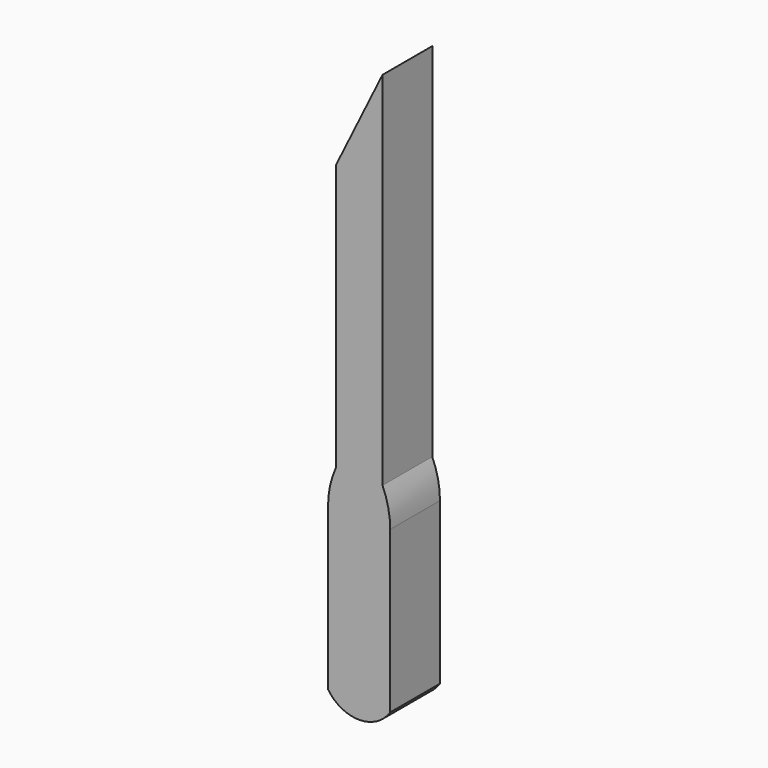
from build123d import *

# Parameters (mm, degrees)
F1_DEPTH    = 3.5
F2_T1_DEPTH = 13.6927447268
F2_T3_DEPTH = 13.6880389421


# Not quite as in the source:
# - a fillet or chamfer that OpenCascade refuses, or shapes differently, is made with other operations: its cross-section is extruded or revolved along the edge and cut away or added


with BuildPart() as f1:
    # F0 (on Front) → F1 (new body)
    with BuildSketch(Plane.XZ):
        with BuildLine():
            Line((-12.9772726037, -35.7954576612), (-16.4772726037, -35.7954576612))
            ThreePointArc((-16.4772726037, -35.7954576612), (-14.7272726037, -36.734376134), (-12.9772726037, -35.7954576612))
        make_face()
        Polygon((-16.0428304225, -9.6928073466), (-16.0428304225, -24.6928073466), (-13.4112946689, -24.6928073466), (-13.4112946689, -4.3468838558), align=None)
        Polygon((-16.4772726037, -24.6928073466), (-16.4772726037, -35.7954576612), (-12.9772726037, -35.7954576612), (-12.9772726037, -24.6928073466), (-13.4112946689, -24.6928073466), (-16.0428304225, -24.6928073466), align=None)
    extrude(amount=F1_DEPTH)

    # F2: fillet of radius 5 on 2 edges, made by hand

    # F2_s2 → F2_t1 (cut)
    with BuildSketch(Plane.XZ.offset(-5.0963723634)):
        with BuildLine():
            ThreePointArc((-16.0428304225, -24.6928073466), (-16.3674560917, -25.6891924599), (-16.4772726037, -26.7313562919))
            Line((-16.4772726037, -26.7313562919), (-16.4772726037, -24.6928073466))
            Line((-16.4772726037, -24.6928073466), (-16.0428304225, -24.6928073466))
        make_face()
    extrude(amount=F2_T1_DEPTH, mode=Mode.SUBTRACT)

    # F2_s4 → F2_t3 (cut)
    with BuildSketch(Plane.XZ.offset(-5.094019471)):
        with BuildLine():
            ThreePointArc((-12.9772726037, -26.730415135), (-13.0869817292, -25.6887553234), (-13.4112946689, -24.6928073466))
            Line((-13.4112946689, -24.6928073466), (-12.9772726037, -24.6928073466))
            Line((-12.9772726037, -24.6928073466), (-12.9772726037, -26.730415135))
        make_face()
    extrude(amount=F2_T3_DEPTH, mode=Mode.SUBTRACT)


solid = f1.part
